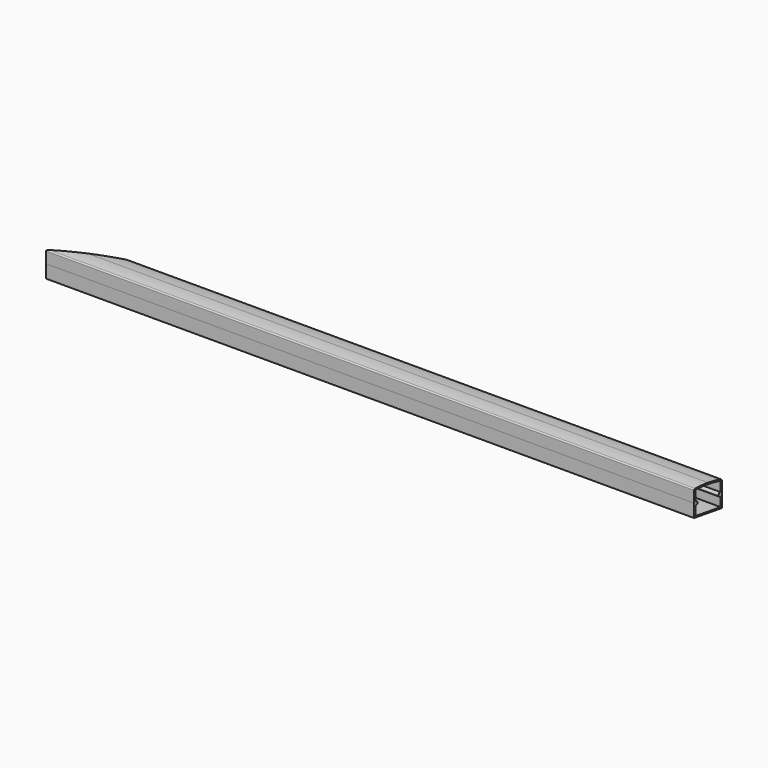
from build123d import *

# Parameters (mm, degrees)
F2_DEPTH      = 1000
F4_DEPTH      = 1000
F8_DEPTH      = 10.001
F8_DEPTH_BACK = 10.001


with BuildPart() as f2:
    # F1 (on Right) → F2 (new body)
    with BuildSketch(Plane.YZ):
        with BuildLine():
            Line((0, -9), (0, -10))
            Line((0, -10), (10, -10))
            Line((10, -10), (10, -0.2))
            Line((10, -0.2), (9, -0.2))
            ThreePointArc((9, -0.2), (8.5, -0.7), (9, -1.2))
            ThreePointArc((9, -1.2), (9.5, -1.7), (9, -2.2))
            Line((9, -2.2), (9, -9))
            Line((9, -9), (0, -9))
        make_face()
    extrude(amount=F2_DEPTH)

    # F5: F2 across plane


with BuildPart() as f4:
    # F3 (on Right) → F4 (new body)
    with BuildSketch(Plane.YZ):
        with BuildLine():
            Line((9, -0.2), (10, -0.2))
            Line((10, -0.2), (10, 8.1663783152))
            ThreePointArc((10, 8.1663783152), (9.7693092582, 8.8052548802), (9.1836734694, 9.1493656277))
            ThreePointArc((9.1836734694, 9.1493656277), (4.6114920912, 9.7868872364), (0, 10))
            Line((0, 10), (0, 9))
            ThreePointArc((0, 9), (4.5192622493, 8.7911494917), (9, 8.1663783152))
            Line((9, 8.1663783152), (9, 0.8))
            ThreePointArc((9, 0.8), (7.5, -0.7), (9, -2.2))
            ThreePointArc((9, -2.2), (9.5, -1.7), (9, -1.2))
            ThreePointArc((9, -1.2), (8.5, -0.7), (9, -0.2))
        make_face()
    extrude(amount=F4_DEPTH)

    # F6: F4 across plane


with BuildPart() as f2_1:
    add(f2.part)
    add(f2.part.mirror(Plane.XZ))


with BuildPart() as f4_1:
    add(f4.part)
    add(f4.part.mirror(Plane.XZ))


with BuildPart() as f8_tool:
    # F7 (on Top) → F8 (new body, two sides)
    with BuildSketch(Plane.XY) as f8_sk:
        Polygon((0, 10), (0, 0), (0, -10), (45.9968509447, 10), align=None)
        Polygon((709.9114181152, 10), (488.8015751816, 10), (484, -10), (1016.9613361359, -10), (1016.9613361359, 10), align=None)
    extrude(amount=F8_DEPTH)
    extrude(f8_sk.sketch, amount=-F8_DEPTH_BACK)


with BuildPart() as f2_2:
    add(f2_1.part)

    # F8: cut by f8_tool
    add(f8_tool.part, mode=Mode.SUBTRACT)


with BuildPart() as f4_2:
    add(f4_1.part)

    # F8: cut by f8_tool
    add(f8_tool.part, mode=Mode.SUBTRACT)


solid = Compound([f2_2.part, f4_2.part])
